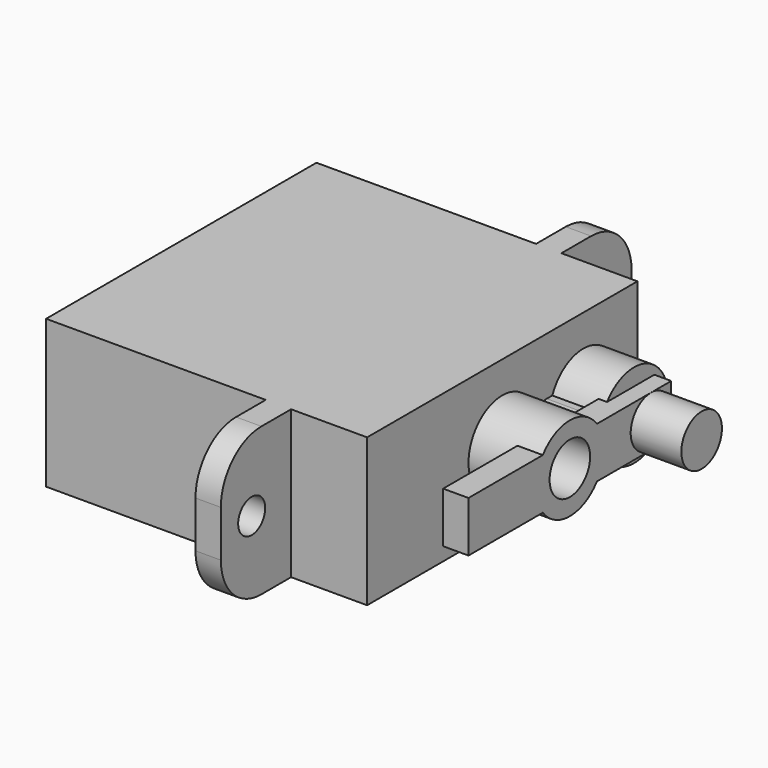
from build123d import *

# Parameters (mm, degrees)
F0_W      = 19
F0_H      = 20
F1_DEPTH  = 4.375
F3_W      = 30.39
F3_H      = 8.75
F3_R      = 1
F4_DEPTH  = 1.5
F6_DEPTH  = 3
F7_R      = 1.5
F8_DEPTH  = 4
F9_R      = 2.5
F10_DEPTH = 4
F12_W     = 15
F12_H     = 3
F13_DEPTH = 1.5
F11_R     = 1.5
F14_DEPTH = 25
F15_R     = 3


with BuildPart() as f1:
    # F0 (on Top) → F1 (new body, symmetric)
    with BuildSketch(Plane.XY):
        with Locations((-9.5, 0)):
            Rectangle(F0_W, F0_H)
    extrude(amount=F1_DEPTH, both=True)

    # F3 (on offset) → F4 (join)
    with BuildSketch(Plane.YZ.offset(-6)):
        Rectangle(F3_W, F3_H)
        with Locations((-12.915, 0)):
            Circle(F3_R, mode=Mode.SUBTRACT)
        with Locations((12.915, 0)):
            Circle(F3_R, mode=Mode.SUBTRACT)
    extrude(amount=F4_DEPTH)

    # F5 (on face) → F6 (join)
    with BuildSketch(Plane.YZ):
        with BuildLine():
            ThreePointArc((3.702386301, -0.9853787547), (6.5029740314, -2.44888079), (8.5, 0))
            ThreePointArc((8.5, 0), (6.5029740314, 2.44888079), (3.702386301, 0.9853787547))
            ThreePointArc((3.702386301, 0.9853787547), (3.5, 0), (3.702386301, -0.9853787547))
        make_face()
        with BuildLine():
            ThreePointArc((3.702386301, -0.9853787547), (3.5, 0), (3.702386301, 0.9853787547))
            Line((3.702386301, 0.9853787547), (3.2885346007, 0.9853787547))
            ThreePointArc((3.2885346007, 0.9853787547), (2.303155846, 0), (3.2885346007, -0.9853787547))
            Line((3.2885346007, -0.9853787547), (3.702386301, -0.9853787547))
        make_face()
    extrude(amount=F6_DEPTH)

    # F7 (on face) → F8 (join)
    with BuildSketch(Plane.YZ.offset(3)):
        with Locations((6, 0)):
            Circle(F7_R)
    extrude(amount=F8_DEPTH)

    # F15
    f15_edges = [f1.edges().sort_by_distance(p)[0] for p in [
        (-5.25, -15.195, -4.375),
        (-5.25, -15.195, 4.375),
        (-5.25, 15.195, -4.375),
        (-5.25, 15.195, 4.375),
    ]]
    fillet(f15_edges, radius=F15_R)


with BuildPart() as f10:
    # F9 (on Right) → F10 (new body)
    with BuildSketch(Plane.YZ):
        Circle(F9_R)
    extrude(amount=F10_DEPTH)

    # F12 (on face) → F13 (join)
    with BuildSketch(Plane.YZ.offset(4)):
        Rectangle(F12_W, F12_H)
    extrude(amount=-F13_DEPTH)

    # F11 (on face) → F14 (cut)
    with BuildSketch(Plane.YZ.offset(4)):
        Circle(F11_R)
    extrude(amount=-F14_DEPTH, mode=Mode.SUBTRACT)


solid = Compound([f1.part, f10.part])
